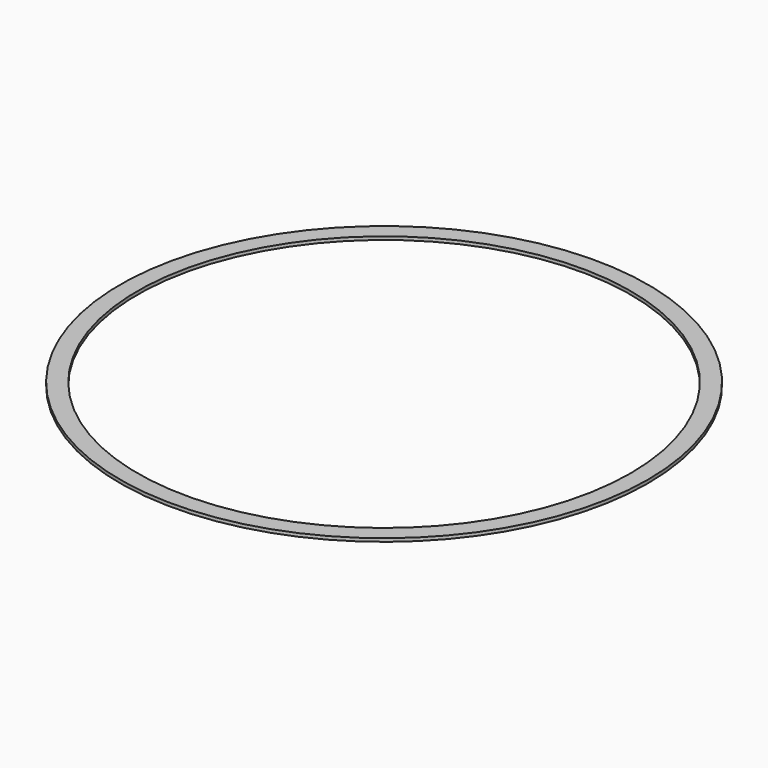
from build123d import *

# Parameters (mm, degrees)
F0_R     = 387.15569
F0_R_2   = 361.75569
F1_DEPTH = 4.7625


# Not quite as in the source:
# - a length typed as a fraction of an inch, garbled in the dataset ("3 / 203.2 mm" for 3/8 in), is restored


with BuildPart() as f1:
    # F0 (on Top) → F1 (new body)
    with BuildSketch(Plane.XY):
        Circle(F0_R)
        Circle(F0_R_2, mode=Mode.SUBTRACT)
    extrude(amount=F1_DEPTH)


solid = f1.part
